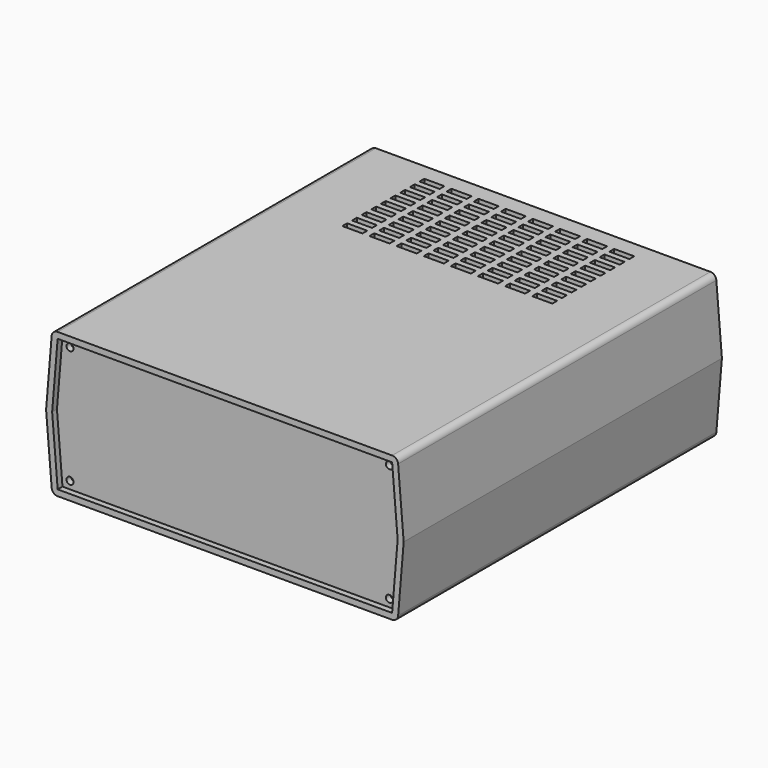
from build123d import *

# Parameters (mm, degrees)
F1_DEPTH     = 198
F2_R         = 3
F4_DEPTH     = 3
F5_T         = 3
F5_T3_DEPTH  = 9
F5_T5_DEPTH  = 39.1143850917
F5_T7_DEPTH  = 39.1143850917
F5_T9_DEPTH  = 172.4792027106
F5_T11_DEPTH = 39.1143850917
F5_T13_DEPTH = 39.1143850917
F6_R         = 1.75
F7_DEPTH     = 25
F8_W         = 10
F8_H         = 3
F9_DEPTH     = 72.001


# Not quite as in the source:
# - a shell that OpenCascade refuses in one call is made with other operations: the cavity is built on its own and cut out


with BuildPart() as f1:
    # F0 (on Front) → F1 (new body)
    with BuildSketch(Plane.XZ):
        Polygon((-86, 36), (-89, 0), (-86, -36), (86, -36), (89, 0), (86, 36), align=None)
    extrude(amount=F1_DEPTH)

    # F2
    f2_edges = [f1.edges().sort_by_distance(p)[0] for p in [
        (86, -99, 36),
        (-86, -99, 36),
        (-86, -99, -36),
        (86, -99, -36),
    ]]
    fillet(f2_edges, radius=F2_R)

    # F3 (on face) → F4 (cut)
    with BuildSketch(Plane.XZ.offset(198)):
        Polygon((-83.2396013553, 33), (-85.9896013553, 0), (-83.2396013553, -33), (83.2396013553, -33), (85.9896013553, 0), (83.2396013553, 33), align=None)
    extrude(amount=-F4_DEPTH, mode=Mode.SUBTRACT)

    # F5: shell of thickness 3, made by hand


with BuildPart() as f5_core1:
    # F5_t2: copy of F1
    add(f1.part)

    # the walls: a layer under each face that stays
    f5_faces = [f5_core1.faces().sort_by_distance(p)[0] for p in [
        (-87.614619315, -99, 16.6245682198),
        (-87.614619315, -99, -16.6245682198),
        (-83.0666666667, -198, -33.6),
        (0, -99, 36),
        (0, -99, -36),
        (87.614619315, -99, 16.6245682198),
        (87.614619315, -99, -16.6245682198),
        (-84.6146013553, -196.5, 16.5),
        (-84.6146013553, -196.5, -16.5),
        (0, -196.5, -33),
        (84.6146013553, -196.5, -16.5),
        (84.6146013553, -196.5, 16.5),
        (0, -196.5, 33),
        (0, -195, 0),
    ]]
    thicken(f5_faces, amount=-F5_T, mode=Mode.SUBTRACT)

    # F5_s4 → F5_t3 (cut)
    with BuildSketch(Plane.XZ.offset(192)):
        Polygon((-83.2097049826, 32.9675086356), (-86.22923863, 33.2491364396), (-86, 36), (-83.2396013553, 36), align=None)
        Polygon((-85.9298086098, 0), (-88.97923863, 0.2491364396), (-89, 0), (-88.97923863, -0.2491364396), align=None)
        Polygon((-83.2097049826, -32.9675086356), (-86.22923863, -33.2491364396), (-86, -36), (-83.2396013553, -36), align=None)
        Polygon((83.2097049826, -32.9675086356), (83.2396013553, -36), (86, -36), (86.22923863, -33.2491364396), align=None)
        Polygon((85.9298086098, 0), (88.97923863, -0.2491364396), (89, 0), (88.97923863, 0.2491364396), align=None)
        Polygon((83.2097049826, 32.9675086356), (86.22923863, 33.2491364396), (86, 36), (83.2396013553, 36), align=None)
    extrude(amount=F5_T3_DEPTH, mode=Mode.SUBTRACT)

    # F5_s6 → F5_t5 (cut)
    with BuildSketch(Plane(origin=(2.4061047061, 0, 28.8732564729), x_dir=(0, 1, 0), z_dir=(-0.0830454799, 0, -0.9965457582))):
        Polygon((-195.03, -85.6625724838), (-195, -88.6925724838), (-192, -88.6925724838), (-192, -85.6925724838), align=None)
    extrude(amount=F5_T5_DEPTH, mode=Mode.SUBTRACT)

    # F5_s8 → F5_t7 (cut)
    with BuildSketch(Plane(origin=(-0.842168173, 0, 10.1060180766), x_dir=(0, 1, 0), z_dir=(0.0830454799, 0, -0.9965457582))):
        Polygon((-195.03, -85.6625724838), (-195, -88.6925724838), (-192, -88.6925724838), (-192, -85.6925724838), align=None)
    extrude(amount=F5_T7_DEPTH, mode=Mode.SUBTRACT)

    # F5_s10 → F5_t9 (cut)
    with BuildSketch(Plane.YZ.offset(-86.2396013553)):
        Polygon((-195.03, -32.97), (-195, -36), (-192, -36), (-192, -33), align=None)
        Polygon((-195.03, 32.97), (-195, 36), (-192, 36), (-192, 33), align=None)
    extrude(amount=F5_T9_DEPTH, mode=Mode.SUBTRACT)

    # F5_s12 → F5_t11 (cut)
    with BuildSketch(Plane(origin=(-2.4061047061, 0, -28.8732564729), x_dir=(0, 1, 0), z_dir=(0.0830454799, 0, 0.9965457582))):
        Polygon((-195.03, -85.6625724838), (-195, -88.6925724838), (-192, -88.6925724838), (-192, -85.6925724838), align=None)
    extrude(amount=F5_T11_DEPTH, mode=Mode.SUBTRACT)

    # F5_s14 → F5_t13 (cut)
    with BuildSketch(Plane(origin=(0.842168173, 0, -10.1060180766), x_dir=(0, 1, 0), z_dir=(-0.0830454799, 0, 0.9965457582))):
        Polygon((-195.03, -85.6625724838), (-195, -88.6925724838), (-192, -88.6925724838), (-192, -85.6925724838), align=None)
    extrude(amount=F5_T13_DEPTH, mode=Mode.SUBTRACT)


with BuildPart() as f1_1:
    add(f1.part)

    # what is left inside the walls is the cavity
    f5_cavity = [f5_core1.part.solids().sort_by_distance(p)[0] for p in [
        (0, -128, -32.97),
    ]]
    add(f5_cavity, mode=Mode.SUBTRACT)

    # F6 (on face) → F7 (cut)
    with BuildSketch(Plane.XZ.offset(195)):
        with Locations((-79.5, 29.25)):
            Circle(F6_R)
        with Locations((79.5, 29.25)):
            Circle(F6_R)
        with Locations((79.5, -29.25)):
            Circle(F6_R)
        with Locations((-79.5, -29.25)):
            Circle(F6_R)
    extrude(amount=-F7_DEPTH, mode=Mode.SUBTRACT)

    # F8 (on face) → F9 (cut, through all)
    with BuildSketch(Plane.XY.offset(36)):
        with Locations((-47.5, -57.8)):
            Rectangle(F8_W, F8_H)
        with Locations((-47.5, -51.8)):
            Rectangle(F8_W, F8_H)
        with Locations((-47.5, -45.8)):
            Rectangle(F8_W, F8_H)
        with Locations((-47.5, -39.8)):
            Rectangle(F8_W, F8_H)
        with Locations((-47.5, -33.8)):
            Rectangle(F8_W, F8_H)
        with Locations((-47.5, -27.8)):
            Rectangle(F8_W, F8_H)
        with Locations((-47.5, -21.8)):
            Rectangle(F8_W, F8_H)
        with Locations((-47.5, -15.8)):
            Rectangle(F8_W, F8_H)
        with Locations((-47.5, -9.8)):
            Rectangle(F8_W, F8_H)
        with Locations((-34, -57.8)):
            Rectangle(F8_W, F8_H)
        with Locations((-34, -51.8)):
            Rectangle(F8_W, F8_H)
        with Locations((-34, -45.8)):
            Rectangle(F8_W, F8_H)
        with Locations((-34, -39.8)):
            Rectangle(F8_W, F8_H)
        with Locations((-34, -33.8)):
            Rectangle(F8_W, F8_H)
        with Locations((-34, -27.8)):
            Rectangle(F8_W, F8_H)
        with Locations((-34, -21.8)):
            Rectangle(F8_W, F8_H)
        with Locations((-34, -15.8)):
            Rectangle(F8_W, F8_H)
        with Locations((-34, -9.8)):
            Rectangle(F8_W, F8_H)
        with Locations((-20.5, -57.8)):
            Rectangle(F8_W, F8_H)
        with Locations((-20.5, -51.8)):
            Rectangle(F8_W, F8_H)
        with Locations((-20.5, -45.8)):
            Rectangle(F8_W, F8_H)
        with Locations((-20.5, -39.8)):
            Rectangle(F8_W, F8_H)
        with Locations((-20.5, -33.8)):
            Rectangle(F8_W, F8_H)
        with Locations((-20.5, -27.8)):
            Rectangle(F8_W, F8_H)
        with Locations((-20.5, -21.8)):
            Rectangle(F8_W, F8_H)
        with Locations((-20.5, -15.8)):
            Rectangle(F8_W, F8_H)
        with Locations((-20.5, -9.8)):
            Rectangle(F8_W, F8_H)
        with Locations((-7, -57.8)):
            Rectangle(F8_W, F8_H)
        with Locations((-7, -51.8)):
            Rectangle(F8_W, F8_H)
        with Locations((-7, -45.8)):
            Rectangle(F8_W, F8_H)
        with Locations((-7, -39.8)):
            Rectangle(F8_W, F8_H)
        with Locations((-7, -33.8)):
            Rectangle(F8_W, F8_H)
        with Locations((-7, -27.8)):
            Rectangle(F8_W, F8_H)
        with Locations((-7, -21.8)):
            Rectangle(F8_W, F8_H)
        with Locations((-7, -15.8)):
            Rectangle(F8_W, F8_H)
        with Locations((-7, -9.8)):
            Rectangle(F8_W, F8_H)
        with Locations((6.5, -57.8)):
            Rectangle(F8_W, F8_H)
        with Locations((6.5, -51.8)):
            Rectangle(F8_W, F8_H)
        with Locations((6.5, -45.8)):
            Rectangle(F8_W, F8_H)
        with Locations((6.5, -39.8)):
            Rectangle(F8_W, F8_H)
        with Locations((6.5, -33.8)):
            Rectangle(F8_W, F8_H)
        with Locations((6.5, -27.8)):
            Rectangle(F8_W, F8_H)
        with Locations((6.5, -21.8)):
            Rectangle(F8_W, F8_H)
        with Locations((6.5, -15.8)):
            Rectangle(F8_W, F8_H)
        with Locations((6.5, -9.8)):
            Rectangle(F8_W, F8_H)
        with Locations((20, -57.8)):
            Rectangle(F8_W, F8_H)
        with Locations((20, -51.8)):
            Rectangle(F8_W, F8_H)
        with Locations((20, -45.8)):
            Rectangle(F8_W, F8_H)
        with Locations((20, -39.8)):
            Rectangle(F8_W, F8_H)
        with Locations((20, -33.8)):
            Rectangle(F8_W, F8_H)
        with Locations((20, -27.8)):
            Rectangle(F8_W, F8_H)
        with Locations((20, -21.8)):
            Rectangle(F8_W, F8_H)
        with Locations((20, -15.8)):
            Rectangle(F8_W, F8_H)
        with Locations((20, -9.8)):
            Rectangle(F8_W, F8_H)
        with Locations((33.5, -57.8)):
            Rectangle(F8_W, F8_H)
        with Locations((33.5, -51.8)):
            Rectangle(F8_W, F8_H)
        with Locations((33.5, -45.8)):
            Rectangle(F8_W, F8_H)
        with Locations((33.5, -39.8)):
            Rectangle(F8_W, F8_H)
        with Locations((33.5, -33.8)):
            Rectangle(F8_W, F8_H)
        with Locations((33.5, -27.8)):
            Rectangle(F8_W, F8_H)
        with Locations((33.5, -21.8)):
            Rectangle(F8_W, F8_H)
        with Locations((33.5, -15.8)):
            Rectangle(F8_W, F8_H)
        with Locations((33.5, -9.8)):
            Rectangle(F8_W, F8_H)
        with Locations((47, -57.8)):
            Rectangle(F8_W, F8_H)
        with Locations((47, -51.8)):
            Rectangle(F8_W, F8_H)
        with Locations((47, -45.8)):
            Rectangle(F8_W, F8_H)
        with Locations((47, -39.8)):
            Rectangle(F8_W, F8_H)
        with Locations((47, -33.8)):
            Rectangle(F8_W, F8_H)
        with Locations((47, -27.8)):
            Rectangle(F8_W, F8_H)
        with Locations((47, -21.8)):
            Rectangle(F8_W, F8_H)
        with Locations((47, -15.8)):
            Rectangle(F8_W, F8_H)
        with Locations((47, -9.8)):
            Rectangle(F8_W, F8_H)
    extrude(amount=-F9_DEPTH, mode=Mode.SUBTRACT)


solid = f1_1.part
